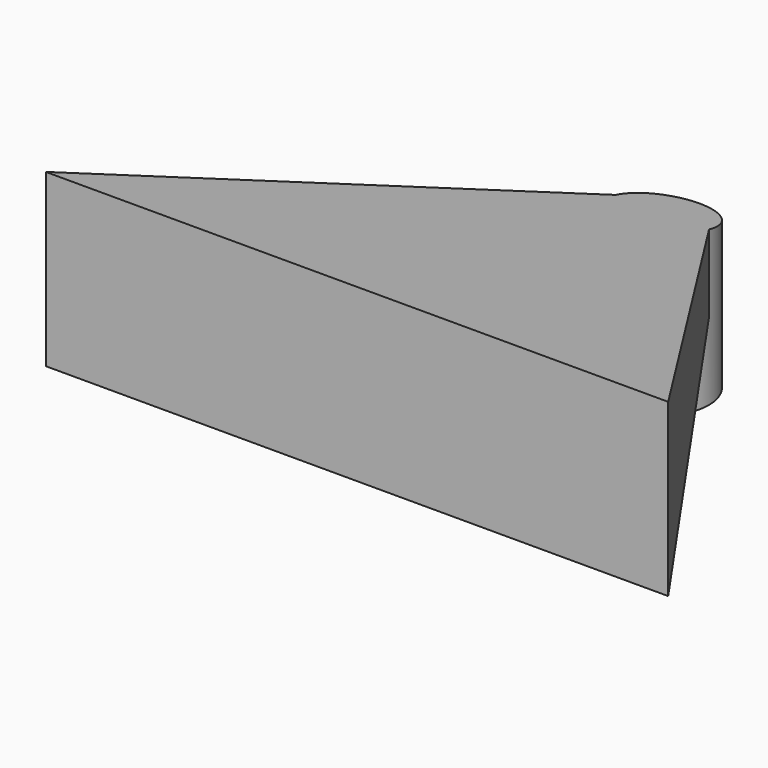
from build123d import *

# Parameters (mm, degrees)
F0_R     = 3
F1_DEPTH = 5
F2_W     = 40
F2_H     = 11
F3_DEPTH = 25
F5_DEPTH = 11.001
F7_DEPTH = 25


with BuildPart() as f1:
    # F0 (on Top) → F1 (new body, symmetric)
    with BuildSketch(Plane.XY):
        Circle(F0_R)
    extrude(amount=F1_DEPTH, both=True)

    # F2 (on Front) → F3 (join)
    with BuildSketch(Plane.XZ):
        with Locations((0.3750487044, 5.5)):
            Rectangle(F2_W, F2_H)
    extrude(amount=F3_DEPTH)

    # F4 (on Top) → F5 (cut, through all)
    with BuildSketch(Plane.XY):
        Polygon((-19.9439544231, -25.4493262619), (-3.0048058834, 0), (-26.9990675151, 2.6770541444), align=None)
        Polygon((32.6401479542, 2.6770541444), (3.0086771585, 0), (20.6934921443, -25.4493262619), align=None)
    extrude(amount=F5_DEPTH, mode=Mode.SUBTRACT)


with BuildPart() as f7:
    # F6 (on Right) → F7 (new body, symmetric)
    with BuildSketch(Plane.YZ):
        Polygon((6.2013822608, 13.6782731861), (-25.7219970226, 11.1731654033), (6.2013822608, 3.444124246), align=None)
    extrude(amount=F7_DEPTH, both=True)


with BuildPart() as f1_1:
    add(f1.part)

    # F8: cut F7
    add(f7.part, mode=Mode.SUBTRACT)


solid = f1_1.part
